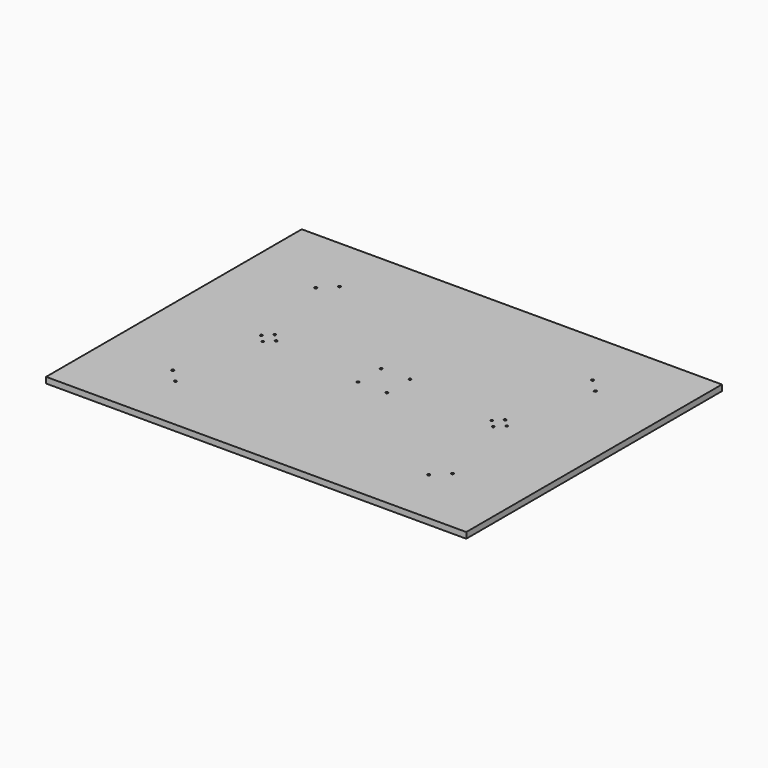
from build123d import *

# Parameters (mm, degrees)
F0_W     = 450.85
F0_H     = 342.9
F1_DEPTH = 6.35
F3_D     = 2.5781
F3_DEPTH = 13.905
F3_TIP   = 0.774539381
F4_D     = 2.5
F5_D     = 2.5
F6_D     = 2.7051
F7_D     = 2.7051


# Not quite as in the source:
# - a feature names something its author has since deleted; it is built from what else it names


with BuildPart() as f1:
    # F0 (on Top) → F1 (new body)
    with BuildSketch(Plane.XY):
        with Locations((-225.425, -171.45)):
            Rectangle(F0_W, F0_H)
    extrude(amount=F1_DEPTH)

    # F3
    with Locations(Plane.XY.offset(6.35)):
        with Locations((-240.925, -155.95), (-209.925, -155.95), (-209.925, -186.95), (-240.925, -186.95)):
            Hole(F3_D / 2, depth=F3_DEPTH)
            with Locations((0, 0, -(F3_DEPTH + F3_TIP / 2))):  # 118° drill point
                Cone(0, F3_D / 2, F3_TIP, mode=Mode.SUBTRACT)

    # F4 (through all)
    with Locations(Plane.XY.offset(6.35)):
        with Locations((-341.075, -171.45), (-357.075, -171.45), (-349.075, -163.45), (-349.075, -179.45)):
            Hole(F4_D / 2)

    # F5 (through all)
    with Locations(Plane.XY.offset(6.35)):
        with Locations((-101.775, -163.45), (-109.775, -171.45), (-101.775, -179.45), (-93.775, -171.45)):
            Hole(F5_D / 2)

    # F6 (through all)
    with Locations(Plane.XY.offset(6.35)):
        with Locations((-361.285, -281.45), (-375.425, -267.31), (-89.565, -281.45), (-75.425, -267.31)):
            Hole(F6_D / 2)

    # F7 (through all)
    with Locations(Plane.XY.offset(6.35)):
        with Locations((-361.285, -61.45), (-375.425, -75.59), (-89.565, -61.45), (-75.425, -75.59)):
            Hole(F7_D / 2)


solid = f1.part
